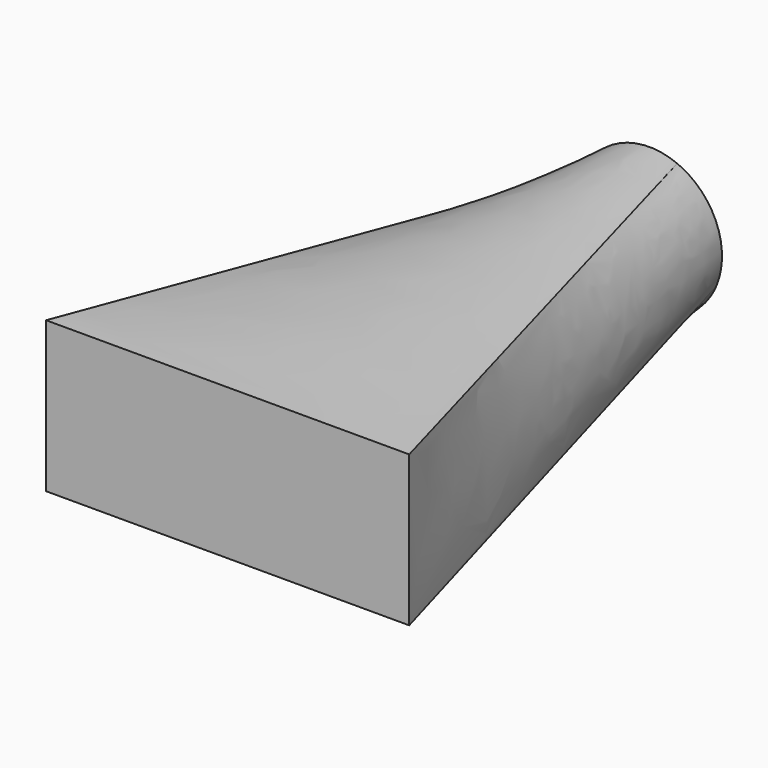
from build123d import *

# Parameters (mm, degrees)
F2_W = 87.4929502606
F2_H = 36.263525486


# Not quite as in the source:
# - the arcs of a loft's sections are written as splines that run evenly, so that the points pair up as in the source's solid


with BuildPart() as f3:
    # F0 (on Front) → F3 section 0
    with BuildSketch(Plane.XZ):
        with BuildLine():
            add(Edge.make_bspline(
                [(-16.1724482445, 6.7030542157), (-16.6111621171, 5.6445699533), (-16.9456161189, 4.5429033874), (-17.3931842646, 2.2954341579), (-17.5062873415, 1.1496870673), (-17.5067960951, -1.1419138849), (-17.3942017592, -2.2877110821), (-16.9476315696, -4.5353788174), (-16.6136667581, -5.6371937776), (-15.7371790672, -7.7545516855), (-15.1946778606, -8.7700422775), (-13.9219555988, -10.6757214811), (-13.1917660141, -11.5658629711), (-11.5717191842, -13.1866292872), (-10.6819019977, -13.9172140368), (-8.7767880909, -15.190782325), (-7.7615384781, -15.733734372), (-6.7030542157, -16.1724482445)],
                knots=[0, 0, 0, 0, 0.125, 0.125, 0.25, 0.25, 0.375, 0.375, 0.5, 0.5, 0.625, 0.625, 0.75, 0.75, 0.875, 0.875, 1, 1, 1, 1], degree=3))
            add(Edge.make_bspline(
                [(-6.7030542157, -16.1724482445), (-5.6445699533, -16.6111621171), (-4.5429033874, -16.9456161189), (-2.2954341579, -17.3931842646), (-1.1496870673, -17.5062873415), (1.1419138849, -17.5067960951), (2.2877110821, -17.3942017592), (4.5353788174, -16.9476315696), (5.6371937776, -16.6136667581), (7.7545516855, -15.7371790672), (8.7700422775, -15.1946778606), (10.6757214811, -13.9219555988), (11.5658629711, -13.1917660141), (13.1866292872, -11.5717191842), (13.9172140368, -10.6819019977), (15.190782325, -8.7767880909), (15.733734372, -7.7615384781), (16.1724482445, -6.7030542157)],
                knots=[0, 0, 0, 0, 0.125, 0.125, 0.25, 0.25, 0.375, 0.375, 0.5, 0.5, 0.625, 0.625, 0.75, 0.75, 0.875, 0.875, 1, 1, 1, 1], degree=3))
            add(Edge.make_bspline(
                [(16.1724482445, -6.7030542157), (16.6111621171, -5.6445699533), (16.9456161189, -4.5429033874), (17.3931842646, -2.2954341579), (17.5062873415, -1.1496870673), (17.5067960951, 1.1419138849), (17.3942017592, 2.2877110821), (16.9476315696, 4.5353788174), (16.6136667581, 5.6371937776), (15.7371790672, 7.7545516855), (15.1946778606, 8.7700422775), (13.9219555988, 10.6757214811), (13.1917660141, 11.5658629711), (11.5717191842, 13.1866292872), (10.6819019977, 13.9172140368), (8.7767880909, 15.190782325), (7.7615384781, 15.733734372), (6.7030542157, 16.1724482445)],
                knots=[0, 0, 0, 0, 0.125, 0.125, 0.25, 0.25, 0.375, 0.375, 0.5, 0.5, 0.625, 0.625, 0.75, 0.75, 0.875, 0.875, 1, 1, 1, 1], degree=3))
            add(Edge.make_bspline(
                [(6.7030542157, 16.1724482445), (5.6445699533, 16.6111621171), (4.5429033874, 16.9456161189), (2.2954341579, 17.3931842646), (1.1496870673, 17.5062873415), (-1.1419138849, 17.5067960951), (-2.2877110821, 17.3942017592), (-4.5353788174, 16.9476315696), (-5.6371937776, 16.6136667581), (-7.7545516855, 15.7371790672), (-8.7700422775, 15.1946778606), (-10.6757214811, 13.9219555988), (-11.5658629711, 13.1917660141), (-13.1866292872, 11.5717191842), (-13.9172140368, 10.6819019977), (-15.190782325, 8.7767880909), (-15.733734372, 7.7615384781), (-16.1724482445, 6.7030542157)],
                knots=[0, 0, 0, 0, 0.125, 0.125, 0.25, 0.25, 0.375, 0.375, 0.5, 0.5, 0.625, 0.625, 0.75, 0.75, 0.875, 0.875, 1, 1, 1, 1], degree=3))
        make_face()
    # F2 (on offset) → F3 section 1
    with BuildSketch(Plane.XZ.offset(127)):
        Rectangle(F2_W, F2_H)
    loft(ruled=True)


solid = f3.part
